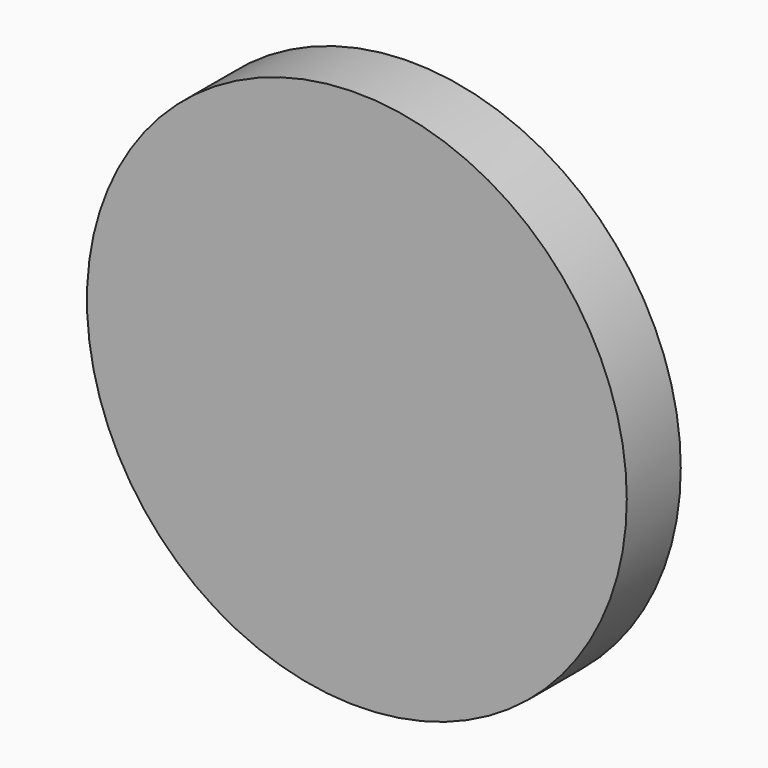
from build123d import *

# Parameters (mm, degrees)
F0_R     = 40
F1_DEPTH = 10


# Not quite as in the source:
# - the program builds the solid bodies; features that only make, move or delete a surface that nothing else refers to are left out


with BuildPart() as f1:
    # F0 (on Front) → F1 (new body)
    with BuildSketch(Plane.XZ):
        Circle(F0_R)
    extrude(amount=F1_DEPTH)


solid = f1.part
